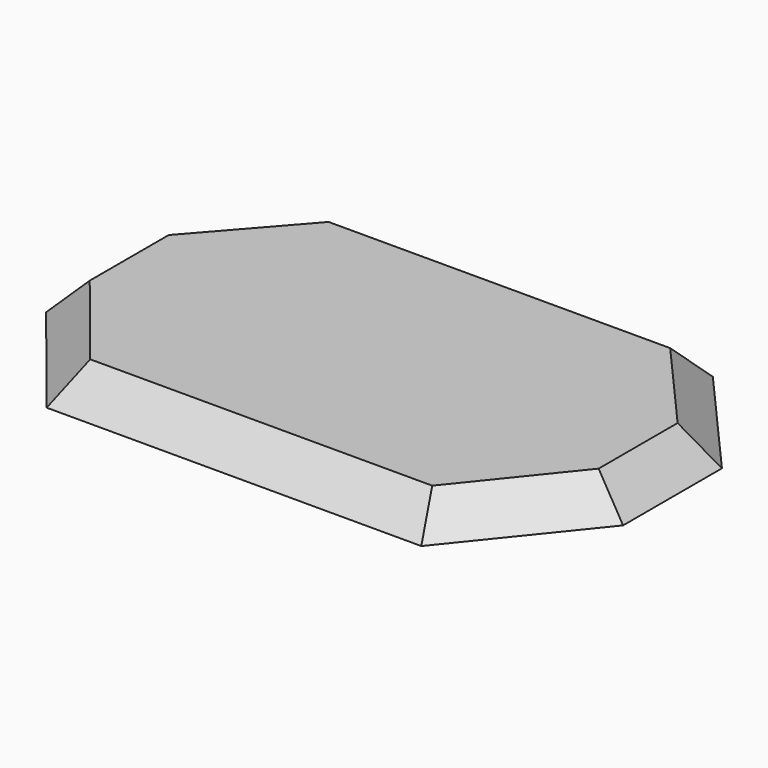
from build123d import *

# Parameters (mm, degrees)
F1_DEPTH     = 3.175
F2_T1_DEPTH  = 39.0408928639
F2_T3_DEPTH  = 42.1701237591
F2_T5_DEPTH  = 62.58572165
F2_T7_DEPTH  = 42.1701213881
F2_T9_DEPTH  = 42.7652991577
F2_T11_DEPTH = 62.8914365267
F2_T13_DEPTH = 42.7652991577


# Not quite as in the source:
# - a fillet or chamfer that OpenCascade refuses, or shapes differently, is made with other operations: its cross-section is extruded or revolved along the edge and cut away or added


with BuildPart() as f1:
    # F0 (on Top) → F1 (new body)
    with BuildSketch(Plane.XY):
        Polygon((28.8131255029, 6.9092694693), (18.2287094494, 18.963740563), (-18.2287130429, 18.963740563), (-28.8131255029, 6.9092694693), (-28.8131255029, -6.0033242369), (-18.3815686845, -18.963740563), (18.3815686845, -18.963740563), (28.8131255029, -6.0033242369), align=None)
    extrude(amount=F1_DEPTH)

    # F2: chamfer of 5.08 on 8 edges, made by hand

    # F2_s2 → F2_t1 (cut)
    with BuildSketch(Plane.XZ.offset(-19.9734190482)):
        Polygon((28.8131255029, -1.905), (23.7331255029, 3.175), (28.8131255029, 3.175), align=None)
        Polygon((-28.8131255029, -1.905), (-23.7331255029, 3.175), (-28.8131255029, 3.175), align=None)
    extrude(amount=F2_T1_DEPTH, mode=Mode.SUBTRACT)

    # F2_s4 → F2_t3 (cut)
    with BuildSketch(Plane(origin=(17.7375583227, -20.2011034897, 0), x_dir=(0, 0, 1), z_dir=(-0.6598012581, 0.7514401506, 0))):
        Polygon((-1.905, 26.210084054), (3.175, 21.130084054), (3.175, 26.210084054), align=None)
    extrude(amount=F2_T3_DEPTH, mode=Mode.SUBTRACT)

    # F2_s6 → F2_t5 (cut)
    with BuildSketch(Plane.YZ.offset(-31.2928626217)):
        Polygon((18.963740563, -1.905), (13.883740563, 3.175), (18.963740563, 3.175), align=None)
    extrude(amount=F2_T5_DEPTH, mode=Mode.SUBTRACT)

    # F2_s8 → F2_t7 (cut)
    with BuildSketch(Plane(origin=(10.0863417988, 11.4872238883, 0), x_dir=(0, 0, 1), z_dir=(-0.6598011316, -0.7514402616, 0))):
        Polygon((-1.905, 26.2100863801), (3.175, 21.1300863801), (3.175, 26.2100863801), align=None)
    extrude(amount=F2_T7_DEPTH, mode=Mode.SUBTRACT)

    # F2_s10 → F2_t9 (cut)
    with BuildSketch(Plane(origin=(-16.5866539058, 20.6076565386, 0), x_dir=(0, 0, 1), z_dir=(0.627009486, -0.7790116202, 0))):
        Polygon((-1.905, 26.2099008264), (3.175, 21.1299008264), (3.175, 26.2099008264), align=None)
    extrude(amount=F2_T9_DEPTH, mode=Mode.SUBTRACT)

    # F2_s12 → F2_t11 (cut)
    with BuildSketch(Plane.YZ.offset(-31.4457182634)):
        Polygon((-18.963740563, -1.905), (-13.883740563, 3.175), (-18.963740563, 3.175), align=None)
    extrude(amount=F2_T11_DEPTH, mode=Mode.SUBTRACT)

    # F2_s14 → F2_t13 (cut)
    with BuildSketch(Plane(origin=(-10.2275943371, -12.7070084487, 0), x_dir=(0, 0, 1), z_dir=(0.627009486, 0.7790116202, 0))):
        Polygon((-1.905, 26.2099008264), (3.175, 21.1299008264), (3.175, 26.2099008264), align=None)
    extrude(amount=F2_T13_DEPTH, mode=Mode.SUBTRACT)


solid = f1.part
